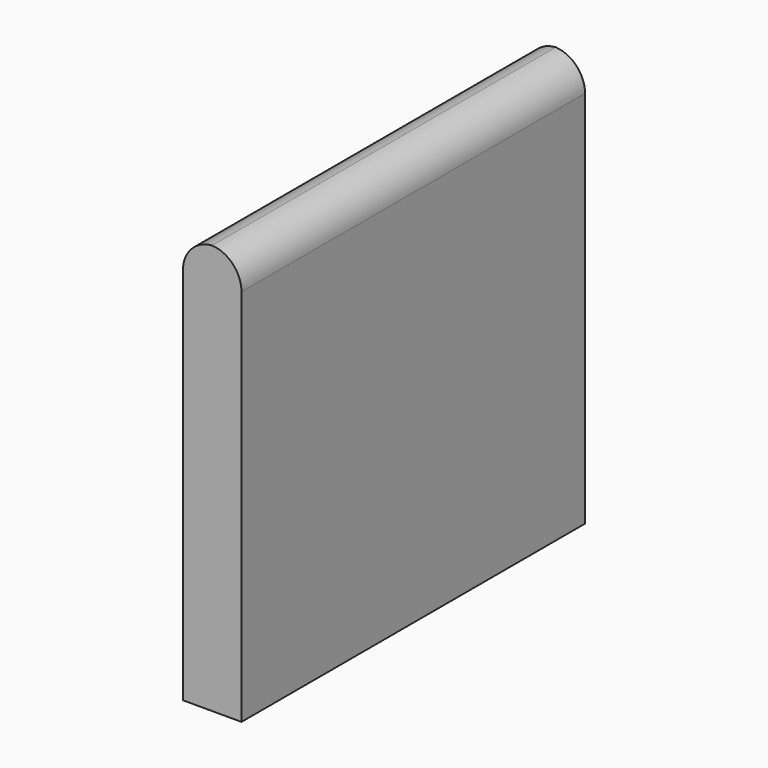
from build123d import *

# Parameters (mm, degrees)
F0_W        = 15
F0_H        = 110
F1_DEPTH    = 105
F2_T1_DEPTH = 150


# Not quite as in the source:
# - a fillet or chamfer that OpenCascade refuses, or shapes differently, is made with other operations: its cross-section is extruded or revolved along the edge and cut away or added


with BuildPart() as f1:
    # F0 (on Top) → F1 (new body)
    with BuildSketch(Plane.XY):
        with Locations((1.6307681799, -0.1918845651)):
            Rectangle(F0_W, F0_H)
    extrude(amount=F1_DEPTH)

    # F2: fillet of radius 8 on 2 edges, made by hand

    # F2_s2 → F2_t1 (cut)
    with BuildSketch(Plane.XZ.offset(-74.8081154349)):
        with BuildLine():
            ThreePointArc((-5.8692318201, 97), (-3.5260860696, 102.6568542495), (2.1307681799, 105))
            Line((2.1307681799, 105), (-5.8692318201, 105))
            Line((-5.8692318201, 105), (-5.8692318201, 97))
        make_face()
        with BuildLine():
            ThreePointArc((9.1307681799, 97), (6.7876224294, 102.6568542495), (1.1307681799, 105))
            Line((1.1307681799, 105), (9.1307681799, 105))
            Line((9.1307681799, 105), (9.1307681799, 97))
        make_face()
    extrude(amount=F2_T1_DEPTH, mode=Mode.SUBTRACT)


solid = f1.part
